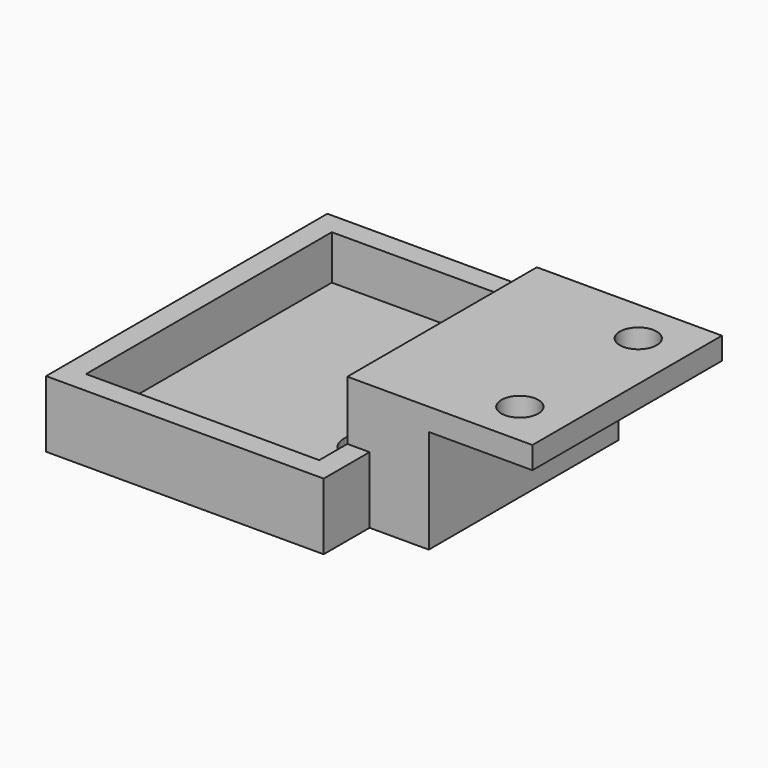
from build123d import *

# Parameters (mm, degrees)
F0_W     = 12.5
F0_H     = 16
F0_R     = 1.25
F1_DEPTH = 1.5
F2_W     = 1.5
F2_H     = 16
F3_DEPTH = 5.5
F5_DEPTH = 3
F4_W     = 1.5
F4_H     = 16
F6_DEPTH = 1.5
F8_DEPTH = 4


# Not quite as in the source:
# - a feature of the source that left no trace in its solid (it failed there, or was rolled back) is left out


with BuildPart() as f1:
    # F0 (on Top) → F1 (new body)
    with BuildSketch(Plane.XY):
        with Locations((-6.25, -8)):
            Rectangle(F0_W, F0_H)
        with Locations((-3.25, -13)):
            Circle(F0_R, mode=Mode.SUBTRACT)
        with Locations((-3.25, -3)):
            Circle(F0_R, mode=Mode.SUBTRACT)
    extrude(amount=F1_DEPTH)

    # F2 (on face) → F3 (join)
    with BuildSketch(Plane(origin=(0, 0, 0), x_dir=(1, 0, 0), z_dir=(0, 0, -1))):
        with Locations((-11.75, 8)):
            Rectangle(F2_W, F2_H)
    extrude(amount=F3_DEPTH)

    # F4 (on face) → F5 (join)
    with BuildSketch(Plane(origin=(0, 0, -5.5), x_dir=(1, 0, 0), z_dir=(0, 0, -1))):
        Polygon((-11, 16), (-11, 19.875), (-29.75, 19.875), (-29.75, -3.875), (-11, -3.875), (-11, 0), (-12.5, 0), (-12.5, -2.375), (-28.25, -2.375), (-28.25, 18.375), (-12.5, 18.375), (-12.5, 16), align=None)
    extrude(amount=-F5_DEPTH)

    # F4 (on face) → F6 (join)
    with BuildSketch(Plane(origin=(0, 0, -5.5), x_dir=(1, 0, 0), z_dir=(0, 0, -1))):
        Polygon((-11, 16), (-11, 19.875), (-29.75, 19.875), (-29.75, -3.875), (-11, -3.875), (-11, 0), (-12.5, 0), (-12.5, -2.375), (-28.25, -2.375), (-28.25, 18.375), (-12.5, 18.375), (-12.5, 16), align=None)
        with Locations((-11.75, 8)):
            Rectangle(F4_W, F4_H)
        Polygon((-12.5, 0), (-12.5, 16), (-12.5, 18.375), (-28.25, 18.375), (-28.25, -2.375), (-12.5, -2.375), align=None)
        with BuildLine():
            Line((-13.375, 11.125), (-13.375, 4.875))
            ThreePointArc((-13.375, 4.875), (-15, 3.25), (-16.625, 4.875))
            Line((-16.625, 4.875), (-16.625, 11.125))
            ThreePointArc((-16.625, 11.125), (-15, 12.75), (-13.375, 11.125))
        make_face(mode=Mode.SUBTRACT)
    extrude(amount=F6_DEPTH)

    # F7 (on face) → F8 (join)
    with BuildSketch(Plane.YZ.offset(-11)):
        Polygon((0, 0), (-16, 0), (-16, -2.5), (-16, -7), (0, -7), (0, -2.5), align=None)
    extrude(amount=F8_DEPTH)


solid = f1.part
